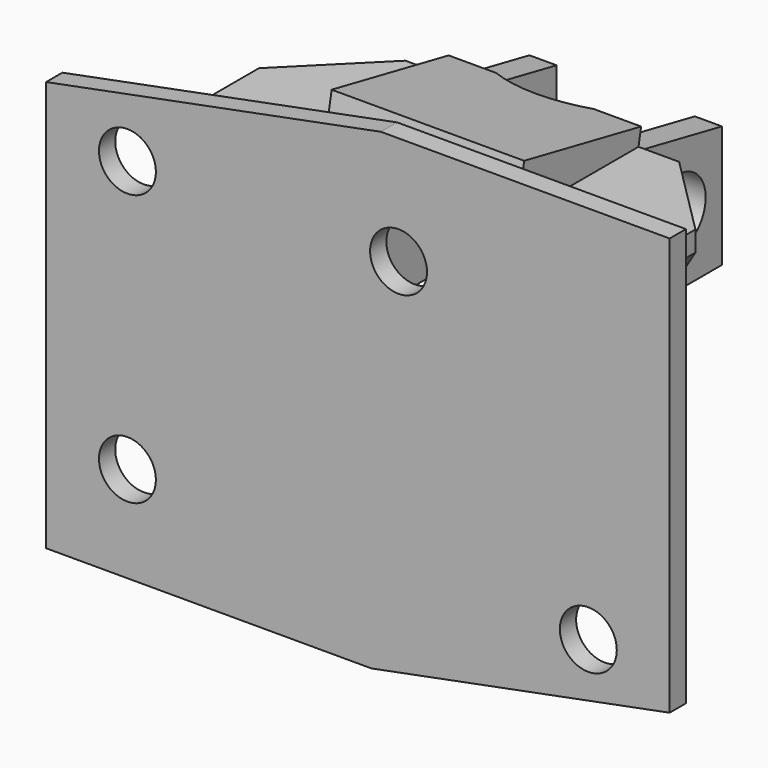
from build123d import *

# Parameters (mm, degrees)
F0_R      = 6.6675
F1_DEPTH  = 4.7625
F2_W      = 6.35
F2_H      = 66.675
F3_DEPTH  = 63.5
F4_R      = 7.9375
F4_W      = 63.5
F4_H      = 25.4
F5_DEPTH  = 87.4548256
F7_DEPTH  = 4.7625
F8_W      = 28.575
F8_H      = 4.7625
F9_REACH  = 92.4701565505
F11_REACH = 103.9121525448
F13_DEPTH = 98.6684645933


with BuildPart() as f1:
    # F0 (on Front) → F1 (new body)
    with BuildSketch(Plane.XZ):
        Polygon((-67.6469967966, 97.79), (-146.05, 82.55), (-146.05, -13.5774645933), (-69.85, -13.5774645933), (0, 0), (0, 97.79), align=None)
        with Locations((-127, 8.89)):
            Circle(F0_R, mode=Mode.SUBTRACT)
        with Locations((-19.05, 8.89)):
            Circle(F0_R, mode=Mode.SUBTRACT)
        with Locations((-127, 72.39)):
            Circle(F0_R, mode=Mode.SUBTRACT)
        with Locations((-63.5, 72.39)):
            Circle(F0_R, mode=Mode.SUBTRACT)
    extrude(amount=F1_DEPTH)

    # F2 (on face) → F3 (join)
    with BuildSketch(Plane(origin=(0, 0, 0), x_dir=(-1, 0, 0), z_dir=(0, 1, 0))):
        with Locations((45.5438256, 58.7375)):
            Rectangle(F2_W, F2_H)
        with Locations((84.2788256, 58.7375)):
            Rectangle(F2_W, F2_H)
    extrude(amount=F3_DEPTH)

    # F4 (on face) → F5 (cut, through all)
    with BuildSketch(Plane(origin=(-87.4538256, 0, 0), x_dir=(0, -1, 0), z_dir=(-1, 0, 0))):
        Polygon((-63.5, 79.375), (0, 92.075), (-63.5, 92.075), align=None)
        with Locations((-50.8, 66.675)):
            Circle(F4_R)
        with Locations((-31.75, 38.1)):
            Rectangle(F4_W, F4_H)
    extrude(amount=-F5_DEPTH, mode=Mode.SUBTRACT)

    # F6 (on face) → F7 (join)
    with BuildSketch(Plane(origin=(0, 17.7067307692, 88.5336538462), x_dir=(1, 0, 0), z_dir=(0, 0.1961161351, 0.9805806757))):
        with BuildLine():
            Line((-87.4538256, -13.2948931428), (-42.3688256, -13.2948931428))
            Line((-42.3688256, -13.2948931428), (-42.3688256, 21.6301068572))
            Line((-42.3688256, 21.6301068572), (-53.4813256, 21.6301068572))
            ThreePointArc((-53.4813256, 21.6301068572), (-64.9113256, 18.9130321535), (-76.3413256, 21.6301068572))
            Line((-76.3413256, 21.6301068572), (-87.4538256, 21.6301068572))
            Line((-87.4538256, 21.6301068572), (-87.4538256, -13.2948931428))
        make_face()
    extrude(amount=F7_DEPTH)

    f9_end = Plane(origin=(-47.9250756, 39.3837971133, 86.6266486207), x_dir=(0, 0.1961161351, 0.9805806757), z_dir=(0, 0.9805806757, -0.1961161351))
    # F8 (on face) → F9 (join, up to a plane its end follows)
    with BuildSketch(Plane(origin=(0, 0, 0), x_dir=(-1, 0, 0), z_dir=(0, 1, 0))):
        with Locations((28.0813256, 82.70875)):
            Rectangle(F8_W, F8_H)
        with Locations((101.7413256, 82.70875)):
            Rectangle(F8_W, F8_H)
    f9_long = extrude(amount=F9_REACH, mode=Mode.PRIVATE)
    add(split(f9_long, bisect_by=f9_end, keep=Keep.BOTTOM, mode=Mode.PRIVATE))

    f11_end = Plane(origin=(-33.5594638675, 38.8165352763, 83.7903394356), x_dir=(0, 0.1961161351, 0.9805806757), z_dir=(0, 0.9805806757, -0.1961161351))
    # F10 (on face) → F11 (join, up to a plane its end follows)
    with BuildSketch(Plane(origin=(0, 0, 0), x_dir=(-1, 0, 0), z_dir=(0, 1, 0))):
        Polygon((20.5290176908, 80.3275), (13.7938256, 80.3275), (42.3688256, 51.7525), (42.3688256, 58.4876920908), align=None)
        Polygon((116.0288256, 80.3275), (109.2936335092, 80.3275), (87.4538256, 58.4876920908), (87.4538256, 51.7525), align=None)
    f11_long = extrude(amount=F11_REACH, mode=Mode.PRIVATE)
    add(split(f11_long, bisect_by=f11_end, keep=Keep.BOTTOM, mode=Mode.PRIVATE))

    # F12 (on face) → F13 (cut, through all)
    with BuildSketch(Plane.XY.offset(85.09)):
        Polygon((-13.7938256, 39.0764673892), (-32.8438256, 39.0764673892), (-13.7938256, 20.0264673892), align=None)
        Polygon((-116.0288256, 20.0264673892), (-96.9788256, 39.0764673892), (-116.0288256, 39.0764673892), align=None)
    extrude(amount=-F13_DEPTH, mode=Mode.SUBTRACT)


solid = f1.part
